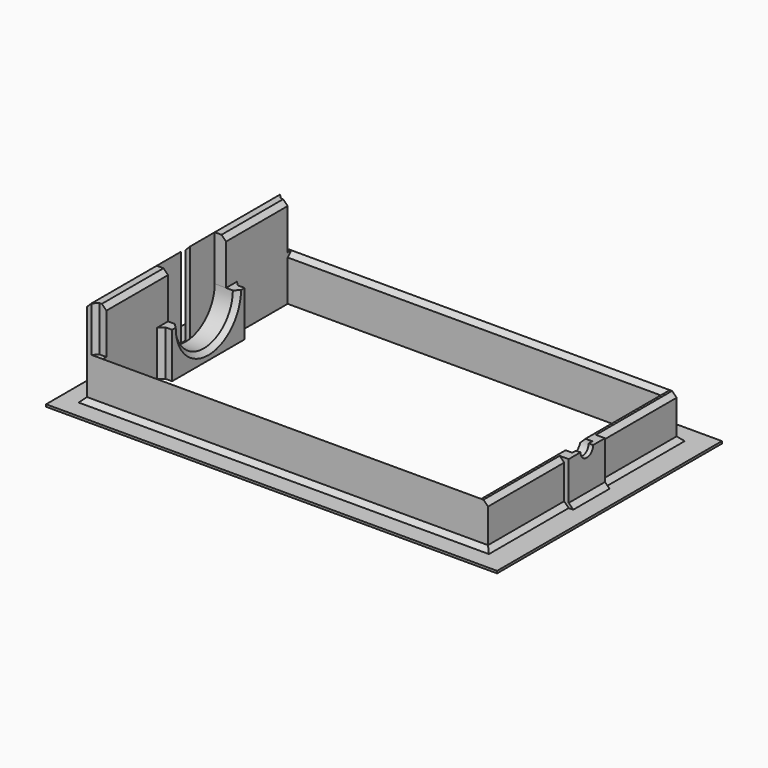
from build123d import *

# Parameters (mm, degrees)
F0_W           = 5
F0_H           = 40
F0_W_2         = 2
F0_H_2         = 20
F1_DEPTH       = 20
F3_DEPTH       = 10
F4_DEPTH       = 175
F6_DEPTH       = 20
F0_H_3         = 49.5
F7_DEPTH       = 40
F8_DEPTH       = 177
F0_W_3         = 199
F0_H_4         = 124
F9_DEPTH       = 1
F10_T1_DEPTH   = 49.5
F10_T3_DEPTH   = 177
F10_T5_DEPTH   = 47.1433659759
F10_T7_DEPTH   = 47.1433659759
F10_T9_DEPTH   = 20
F10_T11_DEPTH  = 20
F10_T13_DEPTH  = 49.5
F10_T15_DEPTH  = 25.1433659759
F10_T20_DEPTH  = 59.7867319519
F10_T25_DEPTH  = 59.7867319519
F10_T31_DEPTH  = 182.1433659759
F10_T35_DEPTH  = 54.6433659759
F10_T42_DEPTH  = 182.1433659759
F10_T46_DEPTH  = 54.6433659759
F10_T53_DEPTH  = 47.1433659759
F10_T57_DEPTH  = 182.1433659759
F10_T64_DEPTH  = 182.1433659759
F10_T68_DEPTH  = 47.1433659759
F10_T71_DEPTH  = 47.1433659759
F10_T73_DEPTH  = 47.1433659759
F10_T75_DEPTH  = 49.6433659759
F10_T77_DEPTH  = 49.6433659759
F10_T79_DEPTH  = 165
F10_T81_DEPTH  = 44.2867319519
F10_T83_DEPTH  = 44.2867319519
F10_T85_DEPTH  = 59.7867319519
F10_T87_DEPTH  = 59.7867319519
F10_T90_ANGLE  = 216.895885655
F10_T95_DEPTH  = 54.7867319519
F10_T100_DEPTH = 170.1433659759
F10_T108_DEPTH = 170.1433659759
F10_T113_DEPTH = 54.7867319519


# Not quite as in the source:
# - a fillet or chamfer that OpenCascade refuses, or shapes differently, is made with other operations: its cross-section is extruded or revolved along the edge and cut away or added


with BuildPart() as f1:
    # F0 (on Top) → F1 (new body)
    with BuildSketch(Plane.XY):
        Polygon((87.5, 52), (-87.5, 52), (-87.5, 2.5), (-87.5, -2.5), (-87.5, -52), (87.5, -52), (87.5, -10), (87.5, 10), align=None)
        Polygon((-82.5, 20), (-82.5, 50), (82.5, 50), (82.5, -50), (-82.5, -50), (-82.5, -20), align=None, mode=Mode.SUBTRACT)
        with Locations((-80, 0)):
            Rectangle(F0_W, F0_H)
        with Locations((88.5, 0)):
            Rectangle(F0_W_2, F0_H_2)
    extrude(amount=F1_DEPTH)

    # F2 (on face) → F3 (cut, through all)
    with BuildSketch(Plane(origin=(-87.5, 0, 0), x_dir=(0, -1, 0), z_dir=(-1, 0, 0))):
        with BuildLine():
            ThreePointArc((-16, 20), (0, 4), (16, 20))
            Line((16, 20), (5.5, 20))
            ThreePointArc((5.5, 20), (0, 14.5), (-5.5, 20))
            Line((-5.5, 20), (-16, 20))
        make_face()
        with BuildLine():
            ThreePointArc((-5.5, 20), (0, 14.5), (5.5, 20))
            Line((5.5, 20), (3.5, 20))
            ThreePointArc((3.5, 20), (0, 16.5), (-3.5, 20))
            Line((-3.5, 20), (-5.5, 20))
        make_face()
    extrude(amount=-F3_DEPTH, mode=Mode.SUBTRACT)

    # F2 (on face) → F4 (cut, through all)
    with BuildSketch(Plane(origin=(-87.5, 0, 0), x_dir=(0, -1, 0), z_dir=(-1, 0, 0))):
        with BuildLine():
            ThreePointArc((-5.5, 20), (0, 14.5), (5.5, 20))
            Line((5.5, 20), (3.5, 20))
            ThreePointArc((3.5, 20), (0, 16.5), (-3.5, 20))
            Line((-3.5, 20), (-5.5, 20))
        make_face()
        with BuildLine():
            ThreePointArc((-3.5, 20), (0, 16.5), (3.5, 20))
            Line((3.5, 20), (-3.5, 20))
        make_face()
    extrude(amount=-F4_DEPTH, mode=Mode.SUBTRACT)

    # F5 (on face) → F6 (join)
    with BuildSketch(Plane.XY.offset(20)):
        Polygon((-82.5, 20), (-82.5, 50), (-87.5, 50), (-87.5, 16), (-82.5, 16), align=None)
        Polygon((-82.5, -16), (-87.5, -16), (-87.5, -50), (-82.5, -50), (-82.5, -20), align=None)
    extrude(amount=F6_DEPTH)

    # F0 (on Top) → F7 (join, through all)
    with BuildSketch(Plane.XY):
        with Locations((-88.5, 27.25)):
            Rectangle(F0_W_2, F0_H_3)
        with Locations((-88.5, -27.25)):
            Rectangle(F0_W_2, F0_H_3)
    extrude(amount=F7_DEPTH)

    # F2 (on face) → F8 (cut, through all)
    with BuildSketch(Plane(origin=(-87.5, 0, 0), x_dir=(0, -1, 0), z_dir=(-1, 0, 0))):
        with BuildLine():
            ThreePointArc((-3.5, 20), (0, 16.5), (3.5, 20))
            Line((3.5, 20), (-3.5, 20))
        make_face()
        with BuildLine():
            Line((-3.5, 20), (3.5, 20))
            ThreePointArc((3.5, 20), (0, 23.5), (-3.5, 20))
        make_face()
    extrude(amount=-F8_DEPTH, mode=Mode.SUBTRACT)

    # F0 (on Top) → F9 (join)
    with BuildSketch(Plane.XY):
        Rectangle(F0_W_3, F0_H_4)
        Polygon((-89.5, 52), (-87.5, 52), (87.5, 52), (87.5, 10), (89.5, 10), (89.5, -10), (87.5, -10), (87.5, -52), (-87.5, -52), (-89.5, -52), (-89.5, -2.5), (-89.5, 2.5), align=None, mode=Mode.SUBTRACT)
    extrude(amount=F9_DEPTH)

    # F10: chamfer of 2 on 23 edges, made by hand

    # F10_s2 → F10_t1 (join)
    with BuildSketch(Plane.XZ.offset(-52)):
        Polygon((-91.5, 1), (-89.5, 3), (-89.5, 1), align=None)
    extrude(amount=F10_T1_DEPTH)

    # F10_s4 → F10_t3 (join)
    with BuildSketch(Plane.YZ.offset(-89.5)):
        Polygon((-54, 1), (-52, 3), (-52, 1), align=None)
        Polygon((52, 3), (54, 1), (52, 1), align=None)
    extrude(amount=F10_T3_DEPTH)

    # F10_s6 → F10_t5 (join)
    with BuildSketch(Plane.XZ.offset(-52)):
        Polygon((89.5, 1), (87.5, 3), (87.5, 1), align=None)
    extrude(amount=F10_T5_DEPTH)

    # F10_s8 → F10_t7 (join)
    with BuildSketch(Plane.XZ.offset(4.8566340241)):
        Polygon((89.5, 1), (87.5, 3), (87.5, 1), align=None)
    extrude(amount=F10_T7_DEPTH)

    # F10_s10 → F10_t9 (join)
    with BuildSketch(Plane.XZ.offset(-10)):
        Polygon((91.5, 1), (89.5, 3), (89.5, 1), align=None)
    extrude(amount=F10_T9_DEPTH)

    # F10_s12 → F10_t11 (join)
    with BuildSketch(Plane.XY):
        Polygon((-82.5, -22), (-80.5, -20), (-82.5, -20), align=None)
        Polygon((-82.5, 22), (-80.5, 20), (-82.5, 20), align=None)
    extrude(amount=F10_T11_DEPTH)

    # F10_s14 → F10_t13 (join)
    with BuildSketch(Plane.XZ.offset(2.5)):
        Polygon((-91.5, 1), (-89.5, 3), (-89.5, 1), align=None)
    extrude(amount=F10_T13_DEPTH)

    # F10_s16 → F10_t15 (join)
    with BuildSketch(Plane.XY.offset(14.8566340241)):
        Polygon((-87.5, 52), (-85.5, 50), (-87.5, 50), align=None)
        Polygon((-87.5, -52), (-85.5, -50), (-87.5, -50), align=None)
    extrude(amount=F10_T15_DEPTH)


with BuildPart() as f10_tool18:
    # F10_s19 → F10_t20 (new body)
    with BuildSketch(Plane.XZ.offset(-57.1433659759)):
        Polygon((-91.5, 1), (-89.5, 3), (-89.5, 1), align=None)
    extrude(amount=F10_T20_DEPTH)

    split(bisect_by=Plane.XZ.offset(2.5), keep=Keep.TOP)


with BuildPart() as f1_1:
    add(f1.part)

    # F10_t17: union F10_tool18
    add(f10_tool18.part)


with BuildPart() as f10_tool23:
    # F10_s24 → F10_t25 (new body)
    with BuildSketch(Plane.XZ.offset(-2.6433659759)):
        Polygon((-91.5, 1), (-89.5, 3), (-89.5, 1), align=None)
    extrude(amount=F10_T25_DEPTH)

    split(bisect_by=Plane.XZ.offset(-2.5), keep=Keep.BOTTOM)


with BuildPart() as f1_2:
    add(f1_1.part)

    # F10_t22: union F10_tool23
    add(f10_tool23.part)


with BuildPart() as f10_tool29:
    # F10_s30 → F10_t31 (new body)
    with BuildSketch(Plane.YZ.offset(87.5)):
        Polygon((52, 3), (54, 1), (52, 1), align=None)
    extrude(amount=-F10_T31_DEPTH)

    split(bisect_by=Plane.YZ.offset(-89.5), keep=Keep.BOTTOM)


with BuildPart() as f10_tool33:
    # F10_s34 → F10_t35 (new body)
    with BuildSketch(Plane.XZ.offset(-57.1433659759)):
        Polygon((-91.5, 1), (-89.5, 3), (-89.5, 1), align=None)
    extrude(amount=F10_T35_DEPTH)

    split(bisect_by=Plane.XZ.offset(-52), keep=Keep.BOTTOM)


with BuildPart() as f10_tool29_1:
    add(f10_tool29.part)

    # F10_t37: intersect F10_tool33
    add(f10_tool33.part, mode=Mode.INTERSECT)


with BuildPart() as f1_3:
    add(f1_2.part)

    # F10_t27: union F10_tool29
    add(f10_tool29_1.part)


with BuildPart() as f10_tool40:
    # F10_s41 → F10_t42 (new body)
    with BuildSketch(Plane.YZ.offset(-94.6433659759)):
        Polygon((-54, 1), (-52, 3), (-52, 1), align=None)
    extrude(amount=F10_T42_DEPTH)

    split(bisect_by=Plane.YZ.offset(-89.5), keep=Keep.BOTTOM)


with BuildPart() as f10_tool44:
    # F10_s45 → F10_t46 (new body)
    with BuildSketch(Plane.XZ.offset(2.5)):
        Polygon((-91.5, 1), (-89.5, 3), (-89.5, 1), align=None)
    extrude(amount=F10_T46_DEPTH)

    split(bisect_by=Plane.XZ.offset(52), keep=Keep.TOP)


with BuildPart() as f10_tool40_1:
    add(f10_tool40.part)

    # F10_t48: intersect F10_tool44
    add(f10_tool44.part, mode=Mode.INTERSECT)


with BuildPart() as f1_4:
    add(f1_3.part)

    # F10_t38: union F10_tool40
    add(f10_tool40_1.part)


with BuildPart() as f10_tool51:
    # F10_s52 → F10_t53 (new body)
    with BuildSketch(Plane.XZ.offset(10)):
        Polygon((89.5, 1), (87.5, 3), (87.5, 1), align=None)
    extrude(amount=F10_T53_DEPTH)

    split(bisect_by=Plane.XZ.offset(52), keep=Keep.TOP)


with BuildPart() as f10_tool55:
    # F10_s56 → F10_t57 (new body)
    with BuildSketch(Plane.YZ.offset(-89.5)):
        Polygon((-54, 1), (-52, 3), (-52, 1), align=None)
    extrude(amount=F10_T57_DEPTH)

    split(bisect_by=Plane.YZ.offset(87.5), keep=Keep.TOP)


with BuildPart() as f10_tool51_1:
    add(f10_tool51.part)

    # F10_t59: intersect F10_tool55
    add(f10_tool55.part, mode=Mode.INTERSECT)


with BuildPart() as f1_5:
    add(f1_4.part)

    # F10_t49: union F10_tool51
    add(f10_tool51_1.part)


with BuildPart() as f10_tool62:
    # F10_s63 → F10_t64 (new body)
    with BuildSketch(Plane.YZ.offset(92.6433659759)):
        Polygon((52, 3), (54, 1), (52, 1), align=None)
    extrude(amount=-F10_T64_DEPTH)

    split(bisect_by=Plane.YZ.offset(87.5), keep=Keep.TOP)


with BuildPart() as f10_tool66:
    # F10_s67 → F10_t68 (new body)
    with BuildSketch(Plane.XZ.offset(-57.1433659759)):
        Polygon((89.5, 1), (87.5, 3), (87.5, 1), align=None)
    extrude(amount=F10_T68_DEPTH)

    split(bisect_by=Plane.XZ.offset(-52), keep=Keep.BOTTOM)


with BuildPart() as f10_tool62_1:
    add(f10_tool62.part)

    # F10_t70: intersect F10_tool66
    add(f10_tool66.part, mode=Mode.INTERSECT)


with BuildPart() as f1_6:
    add(f1_5.part)

    # F10_t60: union F10_tool62
    add(f10_tool62_1.part)

    # F10_s72 → F10_t71 (cut)
    with BuildSketch(Plane.XZ.offset(10)):
        Polygon((85.5, 20), (87.5, 18), (87.5, 20), align=None)
    extrude(amount=F10_T71_DEPTH, mode=Mode.SUBTRACT)

    # F10_s74 → F10_t73 (cut)
    with BuildSketch(Plane.XZ.offset(-57.1433659759)):
        Polygon((87.5, 18), (85.5, 20), (87.5, 20), align=None)
    extrude(amount=F10_T73_DEPTH, mode=Mode.SUBTRACT)

    # F10_s76 → F10_t75 (cut)
    with BuildSketch(Plane.XZ.offset(-50)):
        Polygon((82.5, 18), (84.5, 20), (82.5, 20), align=None)
    extrude(amount=F10_T75_DEPTH, mode=Mode.SUBTRACT)

    # F10_s78 → F10_t77 (cut)
    with BuildSketch(Plane.XZ.offset(0.3566340241)):
        Polygon((84.5, 20), (82.5, 18), (82.5, 20), align=None)
    extrude(amount=F10_T77_DEPTH, mode=Mode.SUBTRACT)

    # F10_s80 → F10_t79 (cut)
    with BuildSketch(Plane.YZ.offset(-82.5)):
        Polygon((50, 18), (52, 20), (50, 20), align=None)
        Polygon((-52, 20), (-50, 18), (-50, 20), align=None)
    extrude(amount=F10_T79_DEPTH, mode=Mode.SUBTRACT)

    # F10_s82 → F10_t81 (cut)
    with BuildSketch(Plane.XZ.offset(10.8566340241)):
        Polygon((-84.5, 40), (-82.5, 38), (-82.5, 40), align=None)
    extrude(amount=F10_T81_DEPTH, mode=Mode.SUBTRACT)

    # F10_s84 → F10_t83 (cut)
    with BuildSketch(Plane.XZ.offset(-55.1433659759)):
        Polygon((-82.5, 38), (-84.5, 40), (-82.5, 40), align=None)
    extrude(amount=F10_T83_DEPTH, mode=Mode.SUBTRACT)

    # F10_s86 → F10_t85 (cut)
    with BuildSketch(Plane.XZ.offset(-2.6433659759)):
        Polygon((-87.5, 40), (-89.5, 38), (-89.5, 40), align=None)
    extrude(amount=F10_T85_DEPTH, mode=Mode.SUBTRACT)

    # F10_s88 → F10_t87 (cut)
    with BuildSketch(Plane.XZ.offset(-57.1433659759)):
        Polygon((-87.5, 40), (-89.5, 38), (-89.5, 40), align=None)
    extrude(amount=F10_T87_DEPTH, mode=Mode.SUBTRACT)

    # F10_s89 → F10_t90 (revolve, cut)
    with BuildSketch(Plane(origin=(0, -6.0036279933, 17.9972777192), x_dir=(1, 0, 0), z_dir=(0, -0.316442908, 0.9486115569))):
        Polygon((-77.5, 24.3288581605), (-79.5, 22.3288581605), (-77.5, 22.3288581605), align=None)
    revolve(axis=Axis((-77.5, 0, 20), (-1, 0, 0)), revolution_arc=F10_T90_ANGLE, mode=Mode.SUBTRACT)


with BuildPart() as f10_tool93:
    # F10_s94 → F10_t95 (new body)
    with BuildSketch(Plane.XZ.offset(-55.1433659759)):
        Polygon((82.5, 18), (84.5, 20), (82.5, 20), align=None)
    extrude(amount=F10_T95_DEPTH)

    split(bisect_by=Plane.XZ.offset(-52), keep=Keep.TOP)

    split(bisect_by=Plane.XZ.offset(-50), keep=Keep.BOTTOM)


with BuildPart() as f10_tool98:
    # F10_s99 → F10_t100 (new body)
    with BuildSketch(Plane.YZ.offset(-82.5)):
        Polygon((50, 18), (52, 20), (50, 20), align=None)
    extrude(amount=F10_T100_DEPTH)

    split(bisect_by=Plane.YZ.offset(87.5), keep=Keep.BOTTOM)

    split(bisect_by=Plane.YZ.offset(82.5), keep=Keep.TOP)


with BuildPart() as f10_tool93_1:
    add(f10_tool93.part)

    # F10_t103: intersect F10_tool98
    add(f10_tool98.part, mode=Mode.INTERSECT)


with BuildPart() as f1_7:
    add(f1_6.part)

    # F10_t91: cut F10_tool93
    add(f10_tool93_1.part, mode=Mode.SUBTRACT)


with BuildPart() as f10_tool106:
    # F10_s107 → F10_t108 (new body)
    with BuildSketch(Plane.YZ.offset(87.6433659759)):
        Polygon((-52, 20), (-50, 18), (-50, 20), align=None)
    extrude(amount=-F10_T108_DEPTH)

    split(bisect_by=Plane.YZ.offset(87.5), keep=Keep.BOTTOM)

    split(bisect_by=Plane.YZ.offset(82.5), keep=Keep.TOP)


with BuildPart() as f10_tool111:
    # F10_s112 → F10_t113 (new body)
    with BuildSketch(Plane.XZ.offset(0.3566340241)):
        Polygon((84.5, 20), (82.5, 18), (82.5, 20), align=None)
    extrude(amount=F10_T113_DEPTH)

    split(bisect_by=Plane.XZ.offset(52), keep=Keep.BOTTOM)

    split(bisect_by=Plane.XZ.offset(50), keep=Keep.TOP)


with BuildPart() as f10_tool106_1:
    add(f10_tool106.part)

    # F10_t116: intersect F10_tool111
    add(f10_tool111.part, mode=Mode.INTERSECT)


with BuildPart() as f1_8:
    add(f1_7.part)

    # F10_t104: cut F10_tool106
    add(f10_tool106_1.part, mode=Mode.SUBTRACT)


solid = f1_8.part
